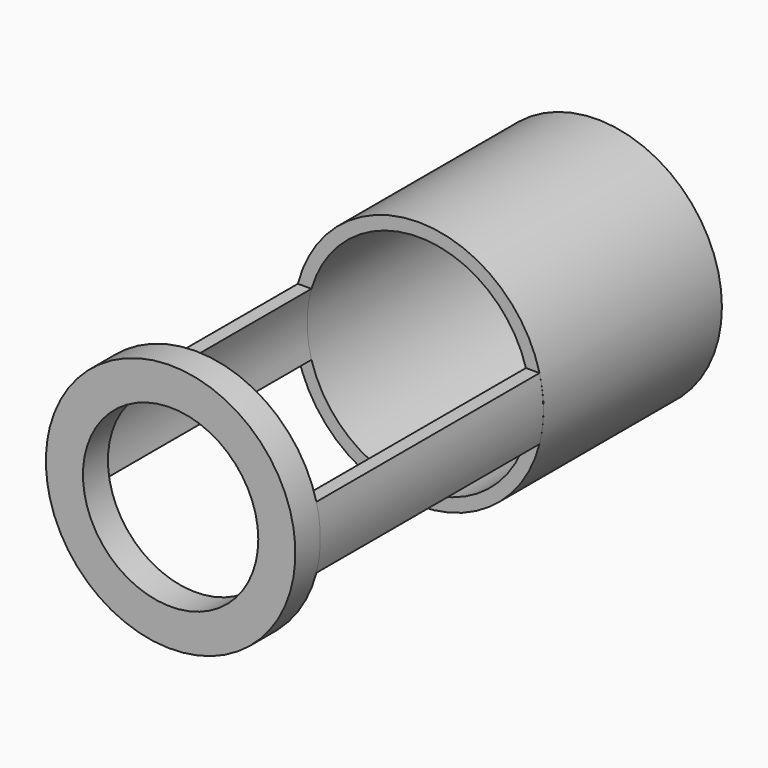
from build123d import *

# Parameters (mm, degrees)
F0_R     = 25.4
F0_R_2   = 22.733
F1_DEPTH = 45.3898
F3_DEPTH = 56.769
F5_R     = 17.8435
F6_DEPTH = 6.35


# Not quite as in the source:
# - a feature of the source that left no trace in its solid (it failed there, or was rolled back) is left out


with BuildPart() as f1:
    # F0 (on Front) → F1 (new body)
    with BuildSketch(Plane.XZ):
        Circle(F0_R)
        Circle(F0_R_2, mode=Mode.SUBTRACT)
    extrude(amount=F1_DEPTH)

    # F2 (on face) → F3 (join)
    with BuildSketch(Plane.XZ.offset(45.3898)):
        with BuildLine():
            ThreePointArc((-21.8250152173, 6.3606603246), (-22.733, 0), (-21.8250152173, -6.3606603246))
            ThreePointArc((-21.8250152173, -6.3606603246), (-22.7199478828, 0), (-21.8250152173, 6.3606603246))
        make_face()
        with BuildLine():
            ThreePointArc((-24.5906892997, 6.3606603246), (-25.3794381847, 0), (-24.5906892997, -6.3606603246))
            Line((-24.5906892997, -6.3606603246), (-21.8250152173, -6.3606603246))
            ThreePointArc((-21.8250152173, -6.3606603246), (-22.733, 0), (-21.8250152173, 6.3606603246))
            Line((-21.8250152173, 6.3606603246), (-24.5906892997, 6.3606603246))
        make_face()
    extrude(amount=F3_DEPTH)

    # F4: F1 across plane


with BuildPart() as f1_1:
    add(f1.part)
    add(f1.part.mirror(Plane.YZ))

    # F5 (on face) → F6 (join)
    with BuildSketch(Plane.XZ.offset(102.1588)):
        with BuildLine():
            Line((-21.8250152173, 6.3606603246), (-24.5906892997, 6.3606603246))
            ThreePointArc((-24.5906892997, 6.3606603246), (-25.3794381847, 0), (-24.5906892997, -6.3606603246))
            Line((-24.5906892997, -6.3606603246), (-21.8250152173, -6.3606603246))
            ThreePointArc((-21.8250152173, -6.3606603246), (-22.7199478828, 0), (-21.8250152173, 6.3606603246))
        make_face()
        with BuildLine():
            ThreePointArc((-24.5906892997, -6.3606603246), (3.2059703513, -25.1968600049), (25.4, 0))
            ThreePointArc((25.4, 0), (3.2059703513, 25.1968600049), (-24.5906892997, 6.3606603246))
            Line((-24.5906892997, 6.3606603246), (-21.8250152173, 6.3606603246))
            ThreePointArc((-21.8250152173, 6.3606603246), (-22.7199478828, 0), (-21.8250152173, -6.3606603246))
            Line((-21.8250152173, -6.3606603246), (-24.5906892997, -6.3606603246))
        make_face()
        Circle(F5_R, mode=Mode.SUBTRACT)
    extrude(amount=F6_DEPTH)


solid = f1_1.part
